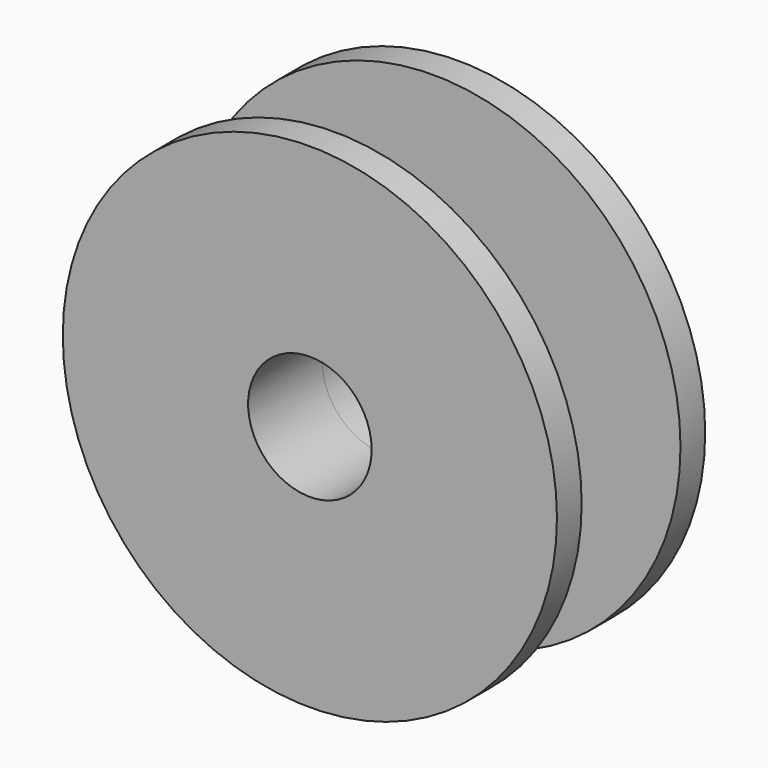
from build123d import *

# Parameters (mm, degrees)
F0_R     = 9.525
F1_DEPTH = 9.525
F2_R     = 25.4
F3_DEPTH = 3.175
F4_R     = 6.35
F5_DEPTH = 12.7


# Not quite as in the source:
# - a length typed as a fraction of an inch, garbled in the dataset ("3 / 203.2 mm" for 3/8 in), is restored


with BuildPart() as f1:
    # F0 (on Front) → F1 (new body)
    with BuildSketch(Plane.XZ):
        Circle(F0_R)
    extrude(amount=F1_DEPTH)

    # F2 (on face) → F3 (join)
    with BuildSketch(Plane.XZ.offset(9.525)):
        Circle(F2_R)
    extrude(amount=-F3_DEPTH)

    # F4 (on face) → F5 (cut, symmetric)
    with BuildSketch(Plane.XZ.offset(9.525)):
        Circle(F4_R)
    extrude(amount=F5_DEPTH, both=True, mode=Mode.SUBTRACT)

    # F6: F1 across plane


with BuildPart() as f1_1:
    add(f1.part)
    add(f1.part.mirror(Plane.XZ))


solid = f1_1.part
